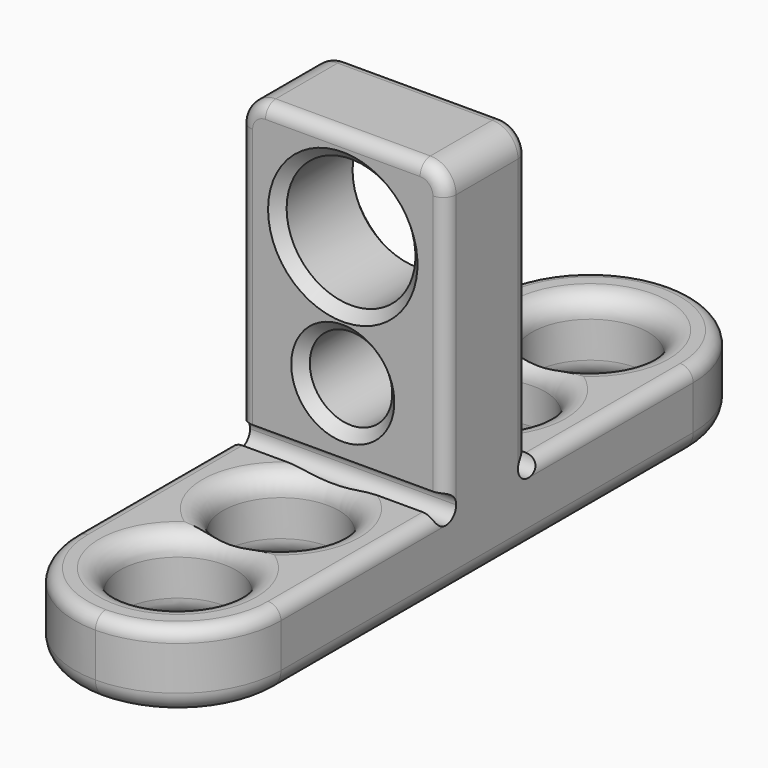
from build123d import *

# Parameters (mm, degrees)
F0_W          = 25.4
F0_H          = 88.9
F1_DEPTH      = 9.525
F2_W          = 25.4
F2_H          = 12.7
F3_DEPTH      = 36.83
F4_R          = 5.08
F4_R_2        = 7.9375
F5_DEPTH      = 50.801
F6_SIZE       = 1.27
F7_R          = 3.175
F8_R          = 12.69999
F9_R          = 7.14375
F10_DEPTH     = 9.526
F12_DEPTH     = 25.401
F13_T1_DEPTH  = 2e-05
F13_T3_DEPTH  = 63.50002
F13_T14_ANGLE = 90
F13_T16_ANGLE = 90
F13_T18_ANGLE = 90
F13_T20_ANGLE = 90
F14_R         = 1.58749


# Not quite as in the source:
# - a fillet or chamfer that OpenCascade refuses, or shapes differently, is made with other operations: its cross-section is extruded or revolved along the edge and cut away or added
# - a fillet or chamfer is up to 0.001 mm smaller than in the source, because OpenCascade refuses the exact size
# - a feature names something its author has since deleted; it is built from what else it names


with BuildPart() as f1:
    # F0 (on Top) → F1 (new body)
    with BuildSketch(Plane.XY):
        Rectangle(F0_W, F0_H)
    extrude(amount=F1_DEPTH)

    # F2 (on face) → F3 (join)
    with BuildSketch(Plane.XY.offset(9.525)):
        Rectangle(F2_W, F2_H)
    extrude(amount=F3_DEPTH)

    # F4 (on face) → F5 (cut, through all)
    with BuildSketch(Plane(origin=(0, 6.35, 0), x_dir=(-1, 0, 0), z_dir=(0, 1, 0))):
        with Locations((0, 19.2405)):
            Circle(F4_R)
        with Locations((0, 35.1155)):
            Circle(F4_R_2)
    extrude(amount=-F5_DEPTH, mode=Mode.SUBTRACT)

    # F6
    f6_edges = [f1.edges().sort_by_distance(p)[0] for p in [
        (5.08, 6.35, 19.2405),
        (-5.08, 0, 19.2405),
        (5.08, -6.35, 19.2405),
        (7.9375, 6.35, 35.1155),
        (-7.9375, 0, 35.1155),
        (7.9375, -6.35, 35.1155),
    ]]
    chamfer(f6_edges, length=F6_SIZE)

    # F7
    f7_edges = [f1.edges().sort_by_distance(p)[0] for p in [
        (-12.7, 0, 46.355),
        (12.7, 0, 46.355),
    ]]
    fillet(f7_edges, radius=F7_R)

    # F8 (radius 12.7 in the source; OpenCascade refuses exactly that, so slightly less here)
    f8_edges = [f1.edges().sort_by_distance(p)[0] for p in [
        (-12.7, 44.45, 4.7625),
        (12.7, 44.45, 4.7625),
        (-12.7, -44.45, 4.7625),
        (12.7, -44.45, 4.7625),
    ]]
    fillet(f8_edges, radius=F8_R)

    # F9 (on face) → F10 (cut, through all)
    with BuildSketch(Plane.XY.offset(9.525)):
        with Locations((0, 31.75)):
            Circle(F9_R)
        with Locations((0, -31.75)):
            Circle(F9_R)
        with Locations((0, 15.875)):
            Circle(F9_R)
        with Locations((0, -15.875)):
            Circle(F9_R)
    extrude(amount=-F10_DEPTH, mode=Mode.SUBTRACT)

    # F11 (on face) → F12 (cut, through all)
    with BuildSketch(Plane.YZ.offset(12.7)):
        with BuildLine():
            ThreePointArc((-4.7625, 9.525), (-5.2274679849, 10.6475320151), (-6.35, 11.1125))
            Line((-6.35, 11.1125), (-6.35, 9.525))
            Line((-6.35, 9.525), (-7.9375, 9.525))
            ThreePointArc((-7.9375, 9.525), (-6.35, 7.9375), (-4.7625, 9.525))
        make_face()
        with BuildLine():
            ThreePointArc((6.35, 11.1125), (5.2274679849, 8.4024679849), (7.9375, 9.525))
            Line((7.9375, 9.525), (6.35, 9.525))
            Line((6.35, 9.525), (6.35, 11.1125))
        make_face()
    extrude(amount=-F12_DEPTH, mode=Mode.SUBTRACT)

    # F13: fillet of radius 2.54 on 20 edges, made by hand

    # F13_s2 → F13_t1 (cut)
    with BuildSketch(Plane.YZ.offset(-1e-05)):
        with BuildLine():
            ThreePointArc((41.91, 0), (43.7060512242, 0.7439487758), (44.45, 2.54))
            Line((44.45, 2.54), (44.45, 0))
            Line((44.45, 0), (41.91, 0))
        make_face()
        with BuildLine():
            ThreePointArc((-41.91, 0), (-43.7060512242, 0.7439487758), (-44.45, 2.54))
            Line((-44.45, 2.54), (-44.45, 0))
            Line((-44.45, 0), (-41.91, 0))
        make_face()
    extrude(amount=F13_T1_DEPTH, mode=Mode.SUBTRACT)

    # F13_s4 → F13_t3 (cut)
    with BuildSketch(Plane.XZ.offset(-31.75001)):
        with BuildLine():
            ThreePointArc((10.16, 0), (11.9560512242, 0.7439487758), (12.7, 2.54))
            Line((12.7, 2.54), (12.7, 0))
            Line((12.7, 0), (10.16, 0))
        make_face()
        with BuildLine():
            ThreePointArc((-12.7, 2.54), (-11.9560512242, 0.7439487758), (-10.16, 0))
            Line((-10.16, 0), (-12.7, 0))
            Line((-12.7, 0), (-12.7, 2.54))
        make_face()
    extrude(amount=F13_T3_DEPTH, mode=Mode.SUBTRACT)

    # F13_s5 → F13_t6 (revolve, cut)
    with BuildSketch(Plane.XZ.offset(-31.75)):
        with BuildLine():
            ThreePointArc((9.68375, 9.525), (7.8876987758, 8.7810512242), (7.14375, 6.985))
            Line((7.14375, 6.985), (7.14375, 9.525))
            Line((7.14375, 9.525), (9.68375, 9.525))
        make_face()
    revolve(axis=Axis((0, 31.75, 9.525), (0, 0, 1)), mode=Mode.SUBTRACT)

    # F13_s7 → F13_t8 (revolve, cut)
    with BuildSketch(Plane.XZ.offset(-31.75)):
        with BuildLine():
            ThreePointArc((9.68375, 0), (7.8876987758, 0.7439487758), (7.14375, 2.54))
            Line((7.14375, 2.54), (7.14375, 0))
            Line((7.14375, 0), (9.68375, 0))
        make_face()
    revolve(axis=Axis((0, 31.75, 0), (0, 0, 1)), mode=Mode.SUBTRACT)

    # F13_s9 → F13_t10 (revolve, cut)
    with BuildSketch(Plane.XZ.offset(31.75)):
        with BuildLine():
            ThreePointArc((9.68375, 9.525), (7.8876987758, 8.7810512242), (7.14375, 6.985))
            Line((7.14375, 6.985), (7.14375, 9.525))
            Line((7.14375, 9.525), (9.68375, 9.525))
        make_face()
    revolve(axis=Axis((0, -31.75, 9.525), (0, 0, 1)), mode=Mode.SUBTRACT)

    # F13_s11 → F13_t12 (revolve, cut)
    with BuildSketch(Plane.XZ.offset(31.75)):
        with BuildLine():
            ThreePointArc((9.68375, 0), (7.8876987758, 0.7439487758), (7.14375, 2.54))
            Line((7.14375, 2.54), (7.14375, 0))
            Line((7.14375, 0), (9.68375, 0))
        make_face()
    revolve(axis=Axis((0, -31.75, 0), (0, 0, 1)), mode=Mode.SUBTRACT)

    # F13_s13 → F13_t14 (revolve, cut)
    with BuildSketch(Plane.XZ.offset(-31.75001)):
        with BuildLine():
            ThreePointArc((10.16, 0), (11.9560512242, 0.7439487758), (12.7, 2.54))
            Line((12.7, 2.54), (12.7, 0))
            Line((12.7, 0), (10.16, 0))
        make_face()
    revolve(axis=Axis((1e-05, 31.75001, 0), (0, 0, 1)), revolution_arc=F13_T14_ANGLE, mode=Mode.SUBTRACT)

    # F13_s15 → F13_t16 (revolve, cut)
    with BuildSketch(Plane.XZ.offset(-31.75001)):
        with BuildLine():
            ThreePointArc((-12.7, 2.54), (-11.9560512242, 0.7439487758), (-10.16, 0))
            Line((-10.16, 0), (-12.7, 0))
            Line((-12.7, 0), (-12.7, 2.54))
        make_face()
    revolve(axis=Axis((-1e-05, 31.75001, 0), (0, 0, -1)), revolution_arc=F13_T16_ANGLE, mode=Mode.SUBTRACT)

    # F13_s17 → F13_t18 (revolve, cut)
    with BuildSketch(Plane.XZ.offset(31.75001)):
        with BuildLine():
            ThreePointArc((10.16, 0), (11.9560512242, 0.7439487758), (12.7, 2.54))
            Line((12.7, 2.54), (12.7, 0))
            Line((12.7, 0), (10.16, 0))
        make_face()
    revolve(axis=Axis((1e-05, -31.75001, 0), (0, 0, -1)), revolution_arc=F13_T18_ANGLE, mode=Mode.SUBTRACT)

    # F13_s19 → F13_t20 (revolve, cut)
    with BuildSketch(Plane.XZ.offset(31.75001)):
        with BuildLine():
            ThreePointArc((-10.16, 0), (-11.9560512242, 0.7439487758), (-12.7, 2.54))
            Line((-12.7, 2.54), (-12.7, 0))
            Line((-12.7, 0), (-10.16, 0))
        make_face()
    revolve(axis=Axis((-1e-05, -31.75001, 0), (0, 0, 1)), revolution_arc=F13_T20_ANGLE, mode=Mode.SUBTRACT)

    # F13_s21 → F13_t22 (revolve, cut)
    with BuildSketch(Plane.XZ.offset(15.875)):
        with BuildLine():
            ThreePointArc((9.68375, 0), (7.8876987758, 0.7439487758), (7.14375, 2.54))
            Line((7.14375, 2.54), (7.14375, 0))
            Line((7.14375, 0), (9.68375, 0))
        make_face()
    revolve(axis=Axis((0, -15.875, 0), (0, 0, 1)), mode=Mode.SUBTRACT)

    # F13_s23 → F13_t24 (revolve, cut)
    with BuildSketch(Plane.XZ.offset(-15.875)):
        with BuildLine():
            ThreePointArc((9.68375, 0), (7.8876987758, 0.7439487758), (7.14375, 2.54))
            Line((7.14375, 2.54), (7.14375, 0))
            Line((7.14375, 0), (9.68375, 0))
        make_face()
    revolve(axis=Axis((0, 15.875, 0), (0, 0, 1)), mode=Mode.SUBTRACT)

    # F13_s25 → F13_t26 (revolve, cut)
    with BuildSketch(Plane.XZ.offset(-15.875)):
        with BuildLine():
            ThreePointArc((9.68375, 9.525), (7.8876987758, 8.7810512242), (7.14375, 6.985))
            Line((7.14375, 6.985), (7.14375, 9.525))
            Line((7.14375, 9.525), (9.68375, 9.525))
        make_face()
    revolve(axis=Axis((0, 15.875, 9.525), (0, 0, 1)), mode=Mode.SUBTRACT)

    # F13_s27 → F13_t28 (revolve, cut)
    with BuildSketch(Plane.XZ.offset(15.875)):
        with BuildLine():
            ThreePointArc((9.68375, 9.525), (7.8876987758, 8.7810512242), (7.14375, 6.985))
            Line((7.14375, 6.985), (7.14375, 9.525))
            Line((7.14375, 9.525), (9.68375, 9.525))
        make_face()
    revolve(axis=Axis((0, -15.875, 9.525), (0, 0, 1)), mode=Mode.SUBTRACT)

    # F14 (radius 1.5875 in the source; OpenCascade refuses exactly that, so slightly less here)
    f14_edges = [f1.edges().sort_by_distance(p)[0] for p in [
        (0, -6.35, 46.355),
        (0, 6.35, 46.355),
        (12.7, 19.843755, 9.525),
        (12.7, -19.843755, 9.525),
    ]]
    fillet(f14_edges, radius=F14_R)


solid = f1.part
